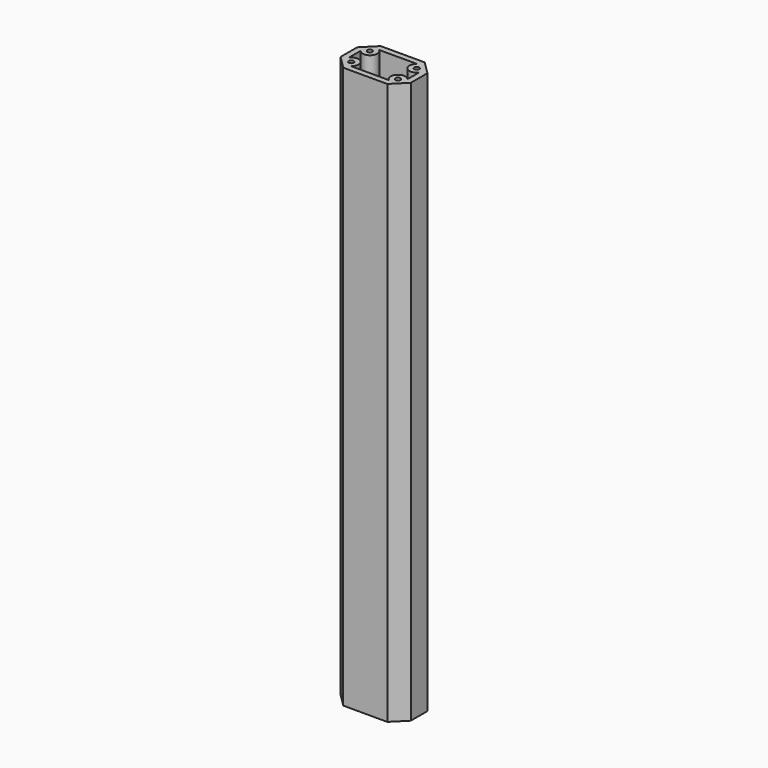
from build123d import *

# Parameters (mm, degrees)
F0_R     = 1.35255
F1_DEPTH = 304.8
F2_T     = 3.175
F3_DEPTH = 3.175
F5_DEPTH = 304.8


# Not quite as in the source:
# - a pattern or mirror of a feature is missing from the dataset's text; its kind, count and spacing are read off the source's solid
# - a shell that OpenCascade refuses in one call is made with other operations: the cavity is built on its own and cut out


with BuildPart() as f1:
    # F0 (on Top) → F1 (new body)
    with BuildSketch(Plane.XY):
        Polygon((11.9626600757, 0), (-11.9626600757, 0), (-19.05, -7.0873399243), (-19.05, -18.3126600757), (-11.9626600757, -25.4), (11.9626600757, -25.4), (19.05, -18.3126600757), (19.05, -7.0873399243), align=None)
        with Locations((-12.7, -19.05)):
            Circle(F0_R, mode=Mode.SUBTRACT)
        with Locations((12.7, -19.05)):
            Circle(F0_R, mode=Mode.SUBTRACT)
        with Locations((-12.7, -6.35)):
            Circle(F0_R, mode=Mode.SUBTRACT)
        with Locations((12.7, -6.35)):
            Circle(F0_R, mode=Mode.SUBTRACT)
    extrude(amount=F1_DEPTH)

    # F2: shell of thickness 3.175, made by hand


with BuildPart() as f2_core1:
    # F2_t2: copy of F1
    add(f1.part)

    # the walls: a layer under each face that stays
    f2_faces = [f2_core1.faces().sort_by_distance(p)[0] for p in [
        (0, 0, 152.4),
        (-15.5063300378, -3.5436699622, 152.4),
        (-19.05, -12.7, 152.4),
        (-15.5063300378, -21.8563300378, 152.4),
        (0, -25.4, 152.4),
        (15.5063300378, -21.8563300378, 152.4),
        (19.05, -12.7, 152.4),
        (15.5063300378, -3.5436699622, 152.4),
        (-14.05255, -19.05, 152.4),
        (11.34745, -19.05, 152.4),
        (-14.05255, -6.35, 152.4),
        (11.34745, -6.35, 152.4),
        (0, -12.7, 0),
    ]]
    thicken(f2_faces, amount=-F2_T, mode=Mode.SUBTRACT)


with BuildPart() as f1_1:
    add(f1.part)

    # what is left inside the walls is the cavity
    f2_cavity = [f2_core1.part.solids().sort_by_distance(p)[0] for p in [
        (0, -3.20675, 204.258333),
    ]]
    add(f2_cavity, mode=Mode.SUBTRACT)

    # F3 (cut, through all): a face of the model
    f3_faces = [f1_1.faces().sort_by_distance(p)[0] for p in [
        (0, -12.7, 3.175),
    ]]
    extrude(f3_faces, amount=-F3_DEPTH, mode=Mode.SUBTRACT)

    # F4 (on face) → F5 (cut, through all)
    with BuildSketch(Plane.XY.offset(304.8)):
        with BuildLine():
            ThreePointArc((15.5063300378, -9.1563300378), (9.8936699622, -9.1563300378), (9.8936699622, -3.5436699622))
            Line((9.8936699622, -3.5436699622), (10.2623399243, -3.175))
            Line((10.2623399243, -3.175), (9.4722943129, -3.175))
            ThreePointArc((9.4722943129, -3.175), (9.4985386928, -9.5514613072), (15.875, -9.5777056871))
            Line((15.875, -9.5777056871), (15.875, -8.7876600757))
            Line((15.875, -8.7876600757), (15.5063300378, -9.1563300378))
        make_face()
        with BuildLine():
            Line((15.875, -16.6123399243), (15.875, -15.8222943129))
            ThreePointArc((15.875, -15.8222943129), (9.4985386928, -15.8485386928), (9.4722943129, -22.225))
            Line((9.4722943129, -22.225), (10.2623399243, -22.225))
            Line((10.2623399243, -22.225), (9.8936699622, -21.8563300378))
            ThreePointArc((9.8936699622, -21.8563300378), (9.8936699622, -16.2436699622), (15.5063300378, -16.2436699622))
            Line((15.5063300378, -16.2436699622), (15.875, -16.6123399243))
        make_face()
    f5 = extrude(amount=-F5_DEPTH, mode=Mode.SUBTRACT)

    # F5_copies: F5 across plane
    add(f5.mirror(Plane(origin=(0, 0, 0), x_dir=(0, 0, -1), z_dir=(-1, 0, 0))), mode=Mode.SUBTRACT)


solid = f1_1.part
